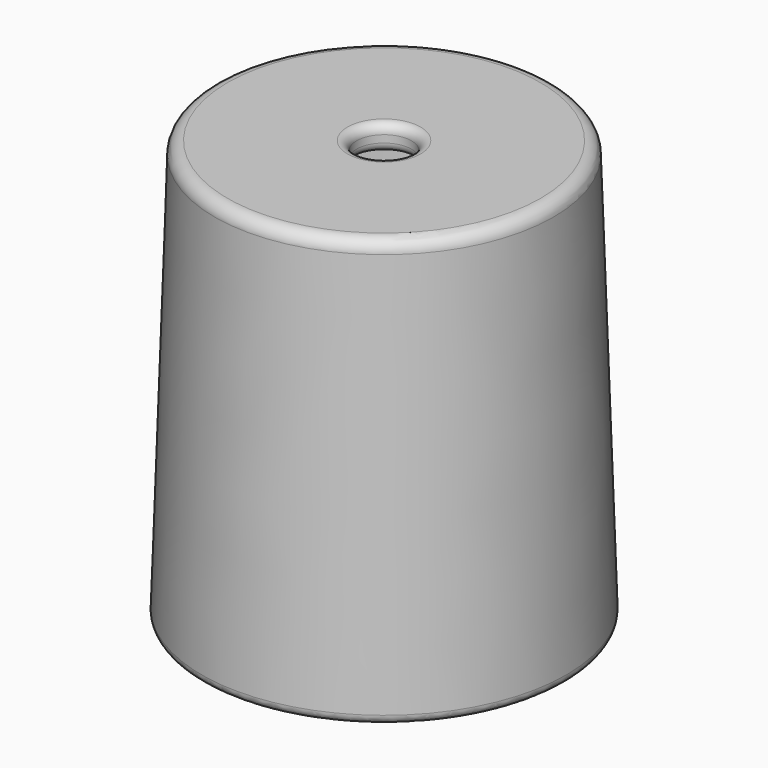
from build123d import *

# Parameters (mm, degrees)
F1_R     = 9.0005312399
F1_R_2   = 8.1515
F4_DEPTH = 3
F7_D     = 3
F7_DEPTH = 12
F7_TIP   = 0.9012909285
F8_R     = 0.7
F9_R     = 0.5


with BuildPart() as f2:
    # F0 (on Front) → F2 (revolve)
    with BuildSketch(Plane.XZ):
        Polygon((0, 21.6), (0, 23), (-9.25, 23), (-10, 0), (-9.0005312399, -0.0325913726), (-8.2820771734, 21.6), align=None)
    revolve(axis=Axis((0, 0, 12.5640318729), (0, 0, -1)))

    # F0 (on Front) → F3 (revolve)
    with BuildSketch(Plane.XZ):
        Polygon((0, 21.6), (0, 23), (-9.25, 23), (-10, 0), (-9.0005312399, -0.0325913726), (-8.2820771734, 21.6), align=None)
    revolve(axis=Axis((0, 0, 12.5640318729), (0, 0, -1)))

    # F1 (on Top) → F4 (join)
    with BuildSketch(Plane.XY):
        Circle(F1_R)
        Circle(F1_R_2, mode=Mode.SUBTRACT)
    extrude(amount=F4_DEPTH)

    # F7
    with Locations(Plane.XY.offset(23)):
        with Locations((0, 0)):
            Hole(F7_D / 2, depth=F7_DEPTH)
            with Locations((0, 0, -(F7_DEPTH + F7_TIP / 2))):  # 118° drill point
                Cone(0, F7_D / 2, F7_TIP, mode=Mode.SUBTRACT)

    # F8
    f8_edges = [f2.edges().sort_by_distance(p)[0] for p in [
        (9.25, 0, 23),
    ]]
    fillet(f8_edges, radius=F8_R)

    # F9
    f9_edges = [f2.edges().sort_by_distance(p)[0] for p in [
        (10, 0, 0),
        (-8.1515, 0, 0),
        (-8.1515, 0, 3),
        (-1.5, 0, 23),
        (-1.5, 0, 21.6),
    ]]
    fillet(f9_edges, radius=F9_R)


solid = f2.part
